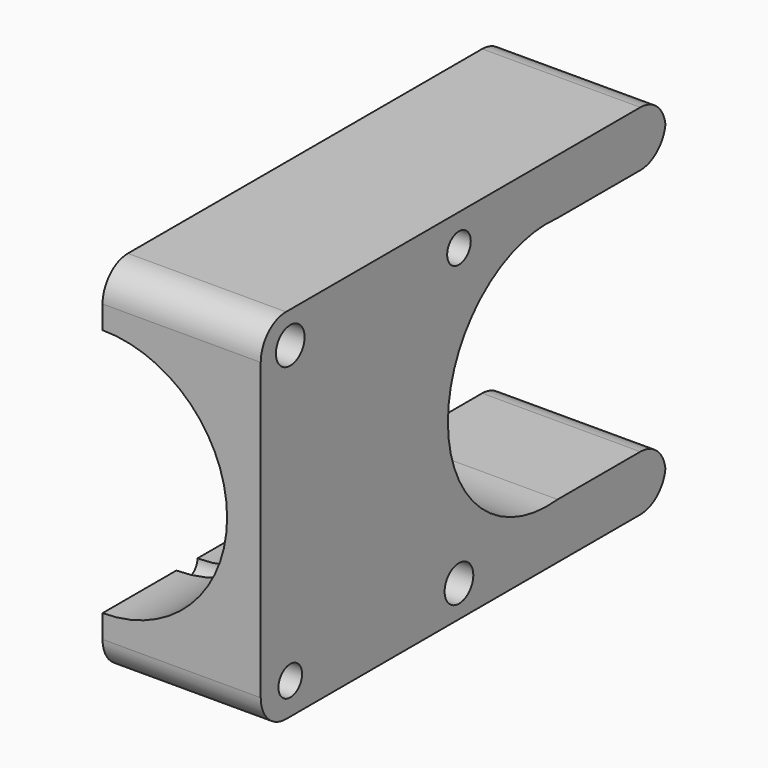
from build123d import *

# Parameters (mm, degrees)
F1_DEPTH      = 10
F1_DEPTH_BACK = 10
F5_DEPTH      = 28
F8_D          = 23.62
F9_D          = 2.8
F9_ON_F2_D    = 2.8
F10_D         = 3.4
F10_ON_F2_D   = 3.4
F7_W          = 14
F7_H          = 23.5
F11_DEPTH     = 25
F12_T1_DEPTH  = 30


# Not quite as in the source:
# - a fillet or chamfer that OpenCascade refuses, or shapes differently, is made with other operations: its cross-section is extruded or revolved along the edge and cut away or added


with BuildPart() as f1:
    # F0 (on Front) → F1 (new body, two sides)
    with BuildSketch(Plane.XZ) as f1_sk:
        with BuildLine():
            Line((15, 17), (0, 17))
            Line((0, 17), (0, 11.81))
            ThreePointArc((0, 11.81), (8.3509310858, 8.3509310858), (11.81, 0))
            ThreePointArc((11.81, 0), (8.3509310858, -8.3509310858), (0, -11.81))
            Line((0, -11.81), (0, -17))
            Line((0, -17), (15, -17))
            Line((15, -17), (15, 17))
        make_face()
    extrude(amount=F1_DEPTH)
    extrude(f1_sk.sketch, amount=-F1_DEPTH_BACK)

    # F2 (on face) → F3 (revolve, cut)
    with BuildSketch(Plane(origin=(0, 0, 0), x_dir=(0, -1, 0), z_dir=(-1, 0, 0))):
        with BuildLine():
            Line((-1.25, -11.81), (1.25, -11.81))
            ThreePointArc((1.25, -11.81), (0, -10.56), (-1.25, -11.81))
        make_face()
        with BuildLine():
            ThreePointArc((-1.25, -11.81), (0, -13.06), (1.25, -11.81))
            Line((1.25, -11.81), (-1.25, -11.81))
        make_face()
    revolve(axis=Axis((0, 0, 0), (0, -1, 0)), mode=Mode.SUBTRACT)

    # F4 (on face) → F5 (join)
    with BuildSketch(Plane(origin=(0, 10, 0), x_dir=(-1, 0, 0), z_dir=(0, 1, 0))):
        with BuildLine():
            Line((0, -11.81), (0, 11.81))
            ThreePointArc((0, 11.81), (-11.81, 0), (0, -11.81))
        make_face()
        with BuildLine():
            Line((0, 17), (-15, 17))
            Line((-15, 17), (-15, -17))
            Line((-15, -17), (0, -17))
            Line((0, -17), (0, -11.81))
            ThreePointArc((0, -11.81), (-11.81, 0), (0, 11.81))
            Line((0, 11.81), (0, 17))
        make_face()
    extrude(amount=F5_DEPTH)

    # F6: union 

    # F8 (through all)
    with Locations(Plane(origin=(0, 0, 0), x_dir=(0, -1, 0), z_dir=(-1, 0, 0))):
        with Locations((-24, 0)):
            Hole(F8_D / 2)

    # F9 (through all)
    with Locations(Plane(origin=(0, 0, 0), x_dir=(0, -1, 0), z_dir=(-1, 0, 0))):
        with Locations((-13.5, 14)):
            Hole(F9_D / 2)

    # F9 on F2 (through all)
    with Locations(Plane(origin=(0, 0, 0), x_dir=(0, -1, 0), z_dir=(-1, 0, 0))):
        with Locations((6.5, -14)):
            Hole(F9_ON_F2_D / 2)

    # F10 (through all)
    with Locations(Plane(origin=(0, 0, 0), x_dir=(0, -1, 0), z_dir=(-1, 0, 0))):
        with Locations((-13.5, -14)):
            Hole(F10_D / 2)

    # F10 on F2 (through all)
    with Locations(Plane(origin=(0, 0, 0), x_dir=(0, -1, 0), z_dir=(-1, 0, 0))):
        with Locations((6.5, 14)):
            Hole(F10_ON_F2_D / 2)

    # F7 (on face) → F11 (cut)
    with BuildSketch(Plane(origin=(0, 0, 0), x_dir=(0, -1, 0), z_dir=(-1, 0, 0))):
        with Locations((-31, 0)):
            Rectangle(F7_W, F7_H)
    extrude(amount=-F11_DEPTH, mode=Mode.SUBTRACT)

    # F12: fillet of radius 3 on 6 edges, made by hand

    # F12_s2 → F12_t1 (cut)
    with BuildSketch(Plane.YZ.offset(-7.5)):
        with BuildLine():
            ThreePointArc((-7, -17), (-9.1213203436, -16.1213203436), (-10, -14))
            Line((-10, -14), (-10, -17))
            Line((-10, -17), (-7, -17))
        make_face()
        with BuildLine():
            ThreePointArc((-7, 17), (-9.1213203436, 16.1213203436), (-10, 14))
            Line((-10, 14), (-10, 17))
            Line((-10, 17), (-7, 17))
        make_face()
        with BuildLine():
            ThreePointArc((38, -14), (37.1213203436, -16.1213203436), (35, -17))
            Line((35, -17), (38, -17))
            Line((38, -17), (38, -14))
        make_face()
        with BuildLine():
            ThreePointArc((35, 17), (37.1213203436, 16.1213203436), (38, 14))
            Line((38, 14), (38, 17))
            Line((38, 17), (35, 17))
        make_face()
        with BuildLine():
            ThreePointArc((35, -11.75), (37.1213203436, -12.6286796564), (38, -14.75))
            Line((38, -14.75), (38, -11.75))
            Line((38, -11.75), (35, -11.75))
        make_face()
        with BuildLine():
            ThreePointArc((38, 14.75), (37.1213203436, 12.6286796564), (35, 11.75))
            Line((35, 11.75), (38, 11.75))
            Line((38, 11.75), (38, 14.75))
        make_face()
    extrude(amount=F12_T1_DEPTH, mode=Mode.SUBTRACT)


solid = f1.part
